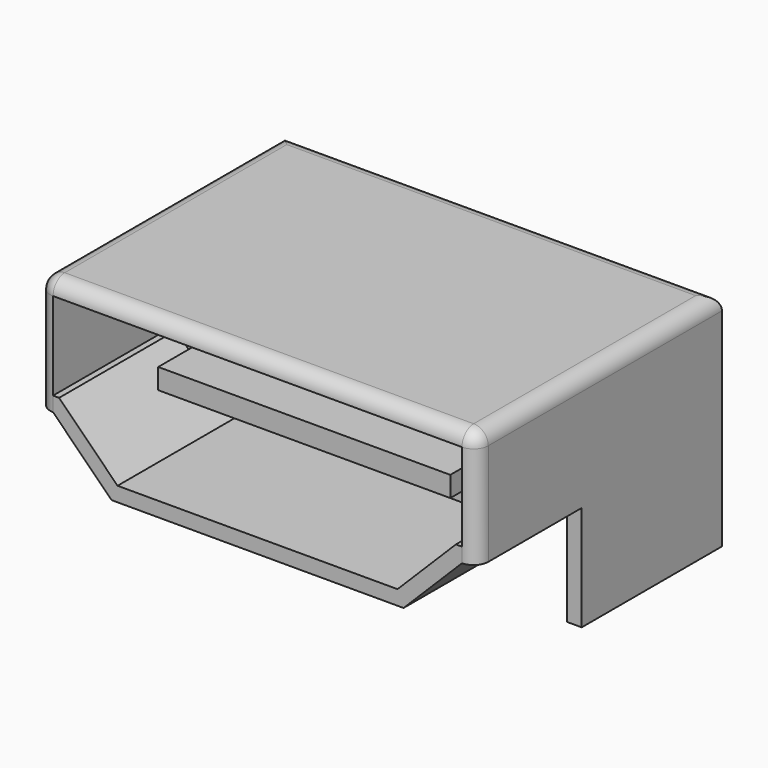
from build123d import *

# Parameters (mm, degrees)
F1_DEPTH = 10.5
F3_DEPTH = 5
F4_W     = 10
F4_H     = 0.7
F5_DEPTH = 3
F6_W     = 0.5
F6_H     = 6
F7_DEPTH = 3.6
F8_R     = 0.49999


# Not quite as in the source:
# - a fillet or chamfer is up to 0.001 mm smaller than in the source, because OpenCascade refuses the exact size


with BuildPart() as f1:
    # F0 (on Front) → F1 (new body)
    with BuildSketch(Plane.XZ):
        Polygon((15, 6), (0, 6), (0, 2), (0.5, 2), (2.5, 0), (12.5, 0), (14.5, 2), (15, 2), align=None)
    extrude(amount=F1_DEPTH)

    # F2 (on face) → F3 (cut)
    with BuildSketch(Plane.XZ.offset(10.5)):
        Polygon((14.5, 5.5), (0.5, 5.5), (0.5, 2.5), (0.7071067812, 2.5), (2.7071067812, 0.5), (12.2928932188, 0.5), (14.2928932188, 2.5), (14.5, 2.5), align=None)
    extrude(amount=-F3_DEPTH, mode=Mode.SUBTRACT)

    # F4 (on face) → F5 (join)
    with BuildSketch(Plane.XZ.offset(5.5)):
        with Locations((7.5, 2.85)):
            Rectangle(F4_W, F4_H)
    extrude(amount=F5_DEPTH)

    # F6 (on face) → F7 (join)
    with BuildSketch(Plane(origin=(0, 0, 2), x_dir=(1, 0, 0), z_dir=(0, 0, -1))):
        with Locations((0.25, 3)):
            Rectangle(F6_W, F6_H)
        with Locations((14.75, 3)):
            Rectangle(F6_W, F6_H)
    extrude(amount=F7_DEPTH)

    # F8 (radius 0.5 in the source; OpenCascade refuses exactly that, so slightly less here)
    f8_edges = [f1.edges().sort_by_distance(p)[0] for p in [
        (0, -5.25, 6),
        (7.5, 0, 6),
        (15, -5.25, 6),
        (7.5, -10.5, 6),
        (0, -10.5, 4),
        (15, -10.5, 4),
    ]]
    fillet(f8_edges, radius=F8_R)


solid = f1.part
